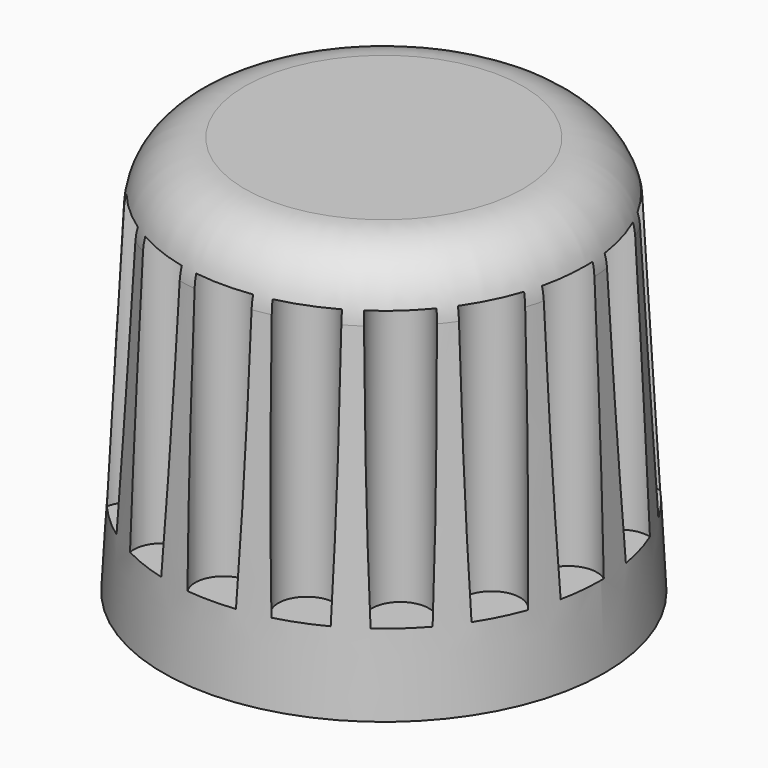
from build123d import *

# Parameters (mm, degrees)
F1_R     = 12.5
F2_DEPTH = 25
F2_TAPER = -3
F3_R     = 1.7835138624
F4_DEPTH = 17
F7_DEPTH = 10


# Not quite as in the source:
# - a fillet or chamfer that OpenCascade refuses, or shapes differently, is made with other operations: its cross-section is extruded or revolved along the edge and cut away or added


with BuildPart() as f2:
    # F1 (on Top) → F2 (new body)
    with BuildSketch(Plane.XY):
        Circle(F1_R)
    extrude(amount=-F2_DEPTH, taper=F2_TAPER)

    # F3 (on offset) → F4 (cut)
    with BuildSketch(Plane.XY.offset(-3)):
        with Locations((0, -12.5270644203)):
            Circle(F3_R)
        with Locations((4.5252976236, -11.6811396879)):
            Circle(F3_R)
        with Locations((8.4394287276, -9.2576123132)):
            Circle(F3_R)
        with Locations((11.2137682175, -5.5837930974)):
            Circle(F3_R)
        with Locations((12.4736261719, -1.155851683)):
            Circle(F3_R)
        with Locations((12.0488517931, 3.4281939061)):
            Circle(F3_R)
        with Locations((9.9968132146, 7.5492429118)):
            Circle(F3_R)
        with Locations((6.5946496173, 10.6507248305)):
            Circle(F3_R)
        with Locations((2.3018420469, 12.3137673431)):
            Circle(F3_R)
        with Locations((-2.3018420469, 12.3137673431)):
            Circle(F3_R)
        with Locations((-6.5946496173, 10.6507248305)):
            Circle(F3_R)
        with Locations((-9.9968132146, 7.5492429118)):
            Circle(F3_R)
        with Locations((-12.0488517931, 3.4281939061)):
            Circle(F3_R)
        with Locations((-12.4736261719, -1.155851683)):
            Circle(F3_R)
        with Locations((-11.2137682175, -5.5837930974)):
            Circle(F3_R)
        with Locations((-8.4394287276, -9.2576123132)):
            Circle(F3_R)
        with Locations((-4.5252976236, -11.6811396879)):
            Circle(F3_R)
    extrude(amount=-F4_DEPTH, mode=Mode.SUBTRACT)

    # F5: fillet of radius 4 on 1 edges, made by hand

    # F5_s1 → F5_t2 (revolve, cut)
    with BuildSketch(Plane.XZ):
        with BuildLine():
            ThreePointArc((12.6986598722, -3.790656175), (11.4575600359, -1.098502516), (8.7041417331, 0))
            Line((8.7041417331, 0), (12.5, 0))
            Line((12.5, 0), (12.6986598722, -3.790656175))
        make_face()
    revolve(axis=Axis((0, 0, 0), (0, 0, -1)), mode=Mode.SUBTRACT)

    # F6 (on face) → F7 (cut)
    with BuildSketch(Plane(origin=(0, 0, -25), x_dir=(1, 0, 0), z_dir=(0, 0, -1))):
        with BuildLine():
            Line((-1.9557109083, -1.3185451265), (1.9557109083, -1.3185451265))
            ThreePointArc((1.9557109083, -1.3185451265), (0, 2.3586789539), (-1.9557109083, -1.3185451265))
        make_face()
    extrude(amount=-F7_DEPTH, mode=Mode.SUBTRACT)


solid = f2.part
